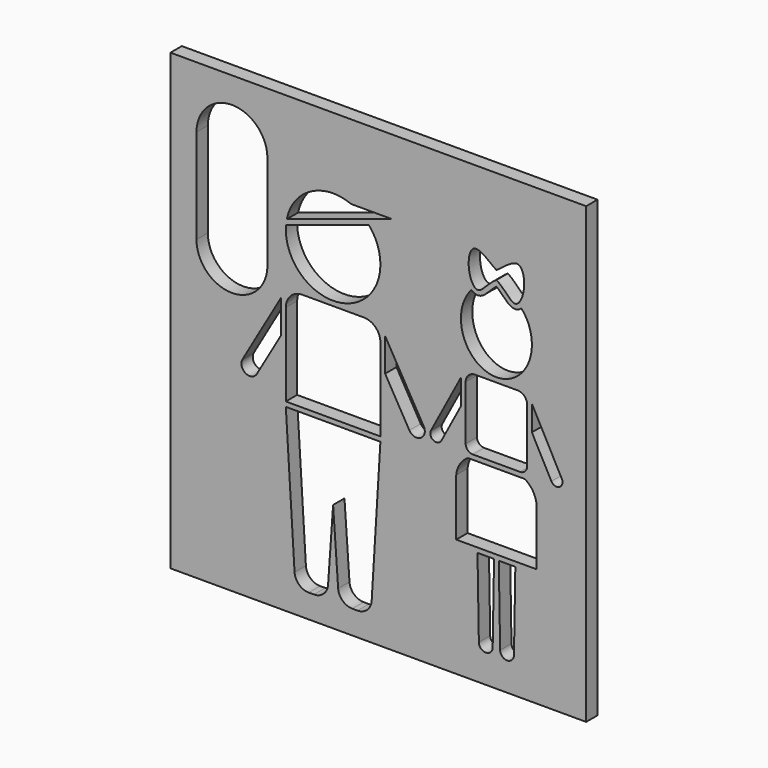
from build123d import *

# Parameters (mm, degrees)
F1_W     = 87.8995961522
F1_H     = 96
F2_DEPTH = 3
F3_DEPTH = 3.001
F5_DEPTH = 3


# Not quite as in the source:
# - ends of sketch curves that miss each other by under 0.0002 mm in the source are joined
# - a feature of the source that left no trace in its solid (it failed there, or was rolled back) is left out
# - the dataset's text gives a spline's control points without its knots; the knots are read off the source's solid


with BuildPart() as f2:
    # F1 (on Front) → F2 (new body)
    with BuildSketch(Plane.XZ):
        with Locations((-15.4397300196, 43)):
            Rectangle(F1_W, F1_H)
    extrude(amount=F2_DEPTH)

    # F0 (on Front) → F3 (cut, through all)
    with BuildSketch(Plane.XZ):
        with BuildLine():
            Line((-12.5, 75.2450460555), (-21.1882912714, 75.2450460555))
            ThreePointArc((-21.1882912714, 75.2450460555), (-29.6990925803, 74.8271472697), (-34.7979589711, 68))
            Line((-34.7979589711, 68), (-12.5, 75.2450460555))
        make_face()
        with BuildLine():
            Line((-18.5, 55), (-31.5, 55))
            ThreePointArc((-31.5, 55), (-33.9748737342, 53.9748737342), (-35, 51.5))
            Line((-35, 51.5), (-35, 34))
            Line((-35, 34), (-15, 34))
            Line((-15, 34), (-15, 51.5))
            ThreePointArc((-15, 51.5), (-16.0251262658, 53.9748737342), (-18.5, 55))
        make_face()
        with BuildLine():
            Line((-17.4689981039, 72.5790584768), (-34.9597820652, 66.8959582652))
            ThreePointArc((-34.9597820652, 66.8959582652), (-21.9098300563, 56.489434837), (-17.4689981039, 72.5790584768))
        make_face()
        with BuildLine():
            Line((-15, 33), (-35, 33))
            Line((-35, 33), (-33.1539197296, 2.8168543814))
            ThreePointArc((-33.1539197296, 2.8168543814), (-32.2150643053, 0.8148870904), (-30.1595153343, 0))
            Line((-30.1595153343, 0), (-29.0562278734, 0))
            ThreePointArc((-29.0562278734, 0), (-27.0102327932, 0.8059388951), (-26.0635357226, 2.7907305788))
            Line((-26.0635357226, 2.7907305788), (-25, 18))
            Line((-25, 18), (-23.9364642774, 2.7907305788))
            ThreePointArc((-23.9364642774, 2.7907305788), (-22.9897672068, 0.8059388951), (-20.9437721266, 0))
            Line((-20.9437721266, 0), (-19.8404846657, 0))
            ThreePointArc((-19.8404846657, 0), (-17.7849356947, 0.8148870904), (-16.8460802704, 2.8168543814))
            Line((-16.8460802704, 2.8168543814), (-15, 33))
        make_face()
        with BuildLine():
            Line((-36, 46), (-36, 53))
            Line((-36, 53), (-44.1550725523, 38.875))
            ThreePointArc((-44.1550725523, 38.875), (-43.5145280957, 36.4844555434), (-41.1239836391, 37.125))
            Line((-41.1239836391, 37.125), (-36, 46))
        make_face()
        with BuildLine():
            Line((-5.8449274477, 38.875), (-14, 53))
            Line((-14, 53), (-14, 46))
            Line((-14, 46), (-8.8760163609, 37.125))
            ThreePointArc((-8.8760163609, 37.125), (-6.4854719043, 36.4844555434), (-5.8449274477, 38.875))
        make_face()
        with BuildLine():
            Line((9.0294127241, 19), (5.5294127241, 19))
            Line((5.5294127241, 19), (5.8180965236, 2.4613162005))
            ThreePointArc((5.8180965236, 2.4613162005), (7.2794127241, 1), (8.7407289245, 2.4613162005))
            Line((8.7407289245, 2.4613162005), (9.0294127241, 19))
        make_face()
        with BuildLine():
            Line((1.0294127241, 20), (9.5294127241, 20))
            Line((9.5294127241, 20), (18.0294127241, 20))
            Line((18.0294127241, 20), (18.0294127241, 32))
            ThreePointArc((18.0294127241, 32), (17.2590555106, 34.2997767416), (15.5294127241, 36))
            Line((15.5294127241, 36), (9.5294127241, 36))
            Line((9.5294127241, 36), (3.5294127241, 36))
            ThreePointArc((3.5294127241, 36), (1.7997699376, 34.2997767416), (1.0294127241, 32))
            Line((1.0294127241, 32), (1.0294127241, 20))
        make_face()
        with BuildLine():
            Line((10.0294127241, 19), (10.3180965236, 2.4613162005))
            ThreePointArc((10.3180965236, 2.4613162005), (11.7794127241, 1), (13.2407289245, 2.4613162005))
            Line((13.2407289245, 2.4613162005), (13.5294127241, 19))
            Line((13.5294127241, 19), (10.0294127241, 19))
        make_face()
        with BuildLine():
            Line((4.5294127241, 37), (9.5294127241, 37))
            Line((9.5294127241, 37), (14.5294127241, 37))
            ThreePointArc((14.5294127241, 37), (15.5900728959, 37.4393398282), (16.0294127241, 38.5))
            Line((16.0294127241, 38.5), (16.0294127241, 50))
            ThreePointArc((16.0294127241, 50), (15.4436262865, 51.4142135624), (14.0294127241, 52))
            Line((14.0294127241, 52), (9.5294127241, 52))
            Line((9.5294127241, 52), (5.0294127241, 52))
            ThreePointArc((5.0294127241, 52), (3.6151991617, 51.4142135624), (3.0294127241, 50))
            Line((3.0294127241, 50), (3.0294127241, 38.5))
            ThreePointArc((3.0294127241, 38.5), (3.4687525523, 37.4393398282), (4.5294127241, 37))
        make_face()
        with BuildLine():
            Line((2.0294127241, 45.1748638295), (2.0294127241, 50.5))
            Line((2.0294127241, 50.5), (-4.3049270994, 38.5868394535))
            ThreePointArc((-4.3049270994, 38.5868394535), (-3.7880820618, 36.8963155089), (-2.0975581173, 37.4131605465))
            Line((-2.0975581173, 37.4131605465), (2.0294127241, 45.1748638295))
        make_face()
        with BuildLine():
            Line((23.3637525476, 38.5868394535), (17.0294127241, 50.5))
            Line((17.0294127241, 50.5), (17.0294127241, 45.1748638295))
            Line((17.0294127241, 45.1748638295), (21.1563835654, 37.4131605465))
            ThreePointArc((21.1563835654, 37.4131605465), (22.84690751, 36.8963155089), (23.3637525476, 38.5868394535))
        make_face()
        with BuildLine():
            add(Edge.make_bspline(
                [(9.5294127241, 69.8736533141), (9.3615824062, 69.7442412015), (9.0301278274, 69.4629383483), (8.5496137897, 68.9981686701), (8.083206253, 68.5185647177), (7.6237511397, 68.0502272834), (7.1532721661, 67.6161990693), (6.7184059809, 67.297838172), (6.2992373245, 67.0929344435), (5.9948825672, 67.0015214228), (5.7262673961, 66.9660619433), (5.4444918801, 66.9622135925), (5.1050027194, 67.0200929358), (4.7428342223, 67.1670834828), (4.4623964247, 67.3465718825), (4.3068278158, 67.4760453145), (4.2454203254, 67.5322172342)],
                knots=[0.0313693059, 0.0313693059, 0.0313693059, 0.0313693059, 0.0625, 0.09375, 0.125, 0.15625, 0.1875, 0.21875, 0.234375, 0.25, 0.2578125, 0.265625, 0.28125, 0.296875, 0.3125, 0.3235896313, 0.3235896313, 0.3235896313, 0.3235896313], degree=3))
            add(Edge.make_bspline(
                [(4.2454203254, 67.5322172342), (-8.6706743361, 53), (9.5294127241, 53), (27.7294997843, 53), (14.8134021156, 67.5322145614)],
                knots=[3.9233560097, 3.9233560097, 3.9233560097, 6.2831853072, 6.2831853072, 8.6430146047, 8.6430146047, 8.6430146047], degree=2, weights=[1, 0.3810037393, 1, 0.3810037393, 1]))
            add(Edge.make_bspline(
                [(9.5294127241, 69.8736533141), (9.6972430419, 69.7442412015), (10.0286976207, 69.4629383483), (10.5092116584, 68.9981686701), (10.9756191951, 68.5185647177), (11.4350743085, 68.0502272834), (11.905553282, 67.6161990693), (12.3404194672, 67.297838172), (12.7595881237, 67.0929344435), (13.063942881, 67.0015214228), (13.332558052, 66.9660619433), (13.614333568, 66.9622135925), (13.9538227287, 67.0200929358), (14.3159912258, 67.1670834828), (14.5964290237, 67.3465718826), (14.7519976327, 67.4760453148), (14.8134021156, 67.5322145614)],
                knots=[0.0313693059, 0.0313693059, 0.0313693059, 0.0313693059, 0.0625, 0.09375, 0.125, 0.15625, 0.1875, 0.21875, 0.234375, 0.25, 0.2578125, 0.265625, 0.28125, 0.296875, 0.3125, 0.3235896313, 0.3235896313, 0.3235896313, 0.3235896313], degree=3))
        make_face()
        with BuildLine():
            add(Edge.make_bspline(
                [(9.5294127241, 71.0850482889), (7.7599830186, 70.0238993272), (5.6413805558, 66.2256414654), (3.1075024949, 71.0756597271), (4.3259185408, 77.6968297412), (8.4780718284, 73.5563934426), (9.5294127241, 72.939933071)],
                knots=[0, 0, 0, 0, 0.2613920824, 0.486624267, 0.7352111742, 1, 1, 1, 1], degree=3))
            add(Edge.make_bspline(
                [(9.5294127241, 71.0850482889), (11.2988424296, 70.0238993272), (13.4174448924, 66.2256414654), (15.9513229533, 71.0756597271), (14.7329069073, 77.6968297412), (10.5807536198, 73.5563934426), (9.5294127241, 72.939933071)],
                knots=[0, 0, 0, 0, 0.2613920824, 0.486624267, 0.7352111742, 1, 1, 1, 1], degree=3))
        make_face()
    extrude(amount=F3_DEPTH, mode=Mode.SUBTRACT)

    # F4 (on face) → F5 (cut, through all)
    with BuildSketch(Plane.XZ.offset(3)):
        with BuildLine():
            Line((-38.8895280957, 58), (-38.8895280957, 78))
            ThreePointArc((-38.8895280957, 78), (-46.3895280957, 85.5), (-53.8895280957, 78))
            Line((-53.8895280957, 78), (-53.8895280957, 58))
            ThreePointArc((-53.8895280957, 58), (-46.3895280957, 50.5), (-38.8895280957, 58))
        make_face()
    extrude(amount=-F5_DEPTH, mode=Mode.SUBTRACT)


solid = f2.part
